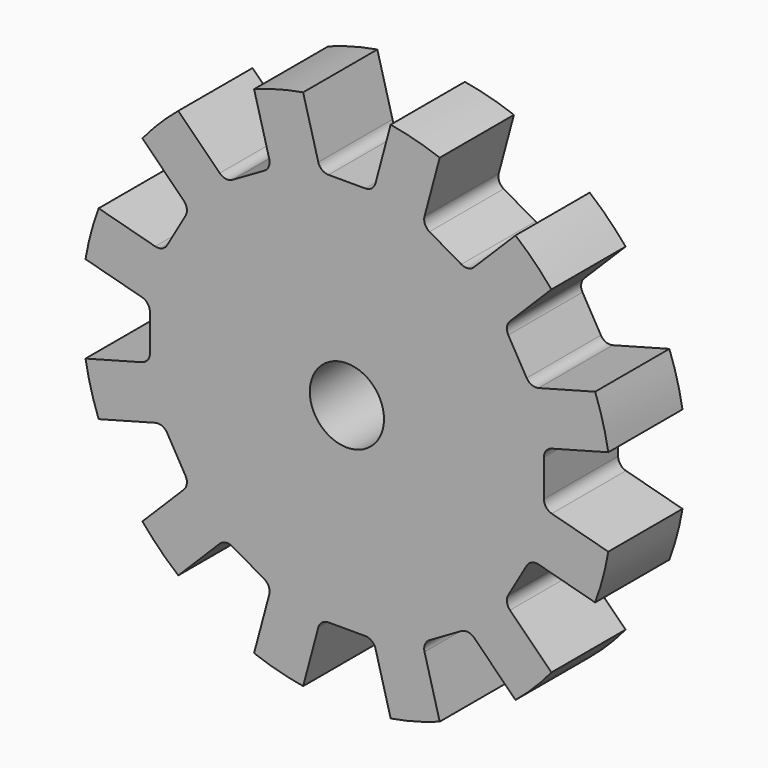
from build123d import *

# Parameters (mm, degrees)
F0_R     = 25.4
F1_DEPTH = 8.89
F3_DEPTH = 25.4
F4_COUNT = 12
F4_ANGLE = 330
F5_R     = 3.556
F6_DEPTH = 25.4


with BuildPart() as f1:
    # F0 (on Front) → F1 (new body)
    with BuildSketch(Plane.XZ):
        Circle(F0_R)
    extrude(amount=F1_DEPTH)

    # F2 (on face) → F3 (cut)
    with BuildSketch(Plane.XZ.offset(8.89)):
        with BuildLine():
            ThreePointArc((1.7603957802, 18.8799073091), (2.3788973921, 19.0898603154), (2.7417764197, 19.6329471593))
            Line((2.7417764197, 19.6329471593), (4.19365, 25.0514131273))
            ThreePointArc((4.19365, 25.0514131274), (0, 25.4), (-4.19365, 25.0514131274))
            Line((-4.19365, 25.0514131273), (-2.7417764197, 19.6329471593))
            ThreePointArc((-2.7417764197, 19.6329471593), (-2.3788973921, 19.0898603154), (-1.7603957802, 18.8799073091))
            Line((-1.7603957802, 18.8799073091), (0, 18.8799073091))
            Line((0, 18.8799073091), (1.7603957802, 18.8799073091))
        make_face()
    f3 = extrude(amount=-F3_DEPTH, mode=Mode.SUBTRACT)

    # F4: F3 ×12 about axis
    f4_axis = Axis((0, 0, 0), (0, 1, 0))
    for i in range(1, F4_COUNT):
        add(f3.rotate(f4_axis, i * F4_ANGLE / (F4_COUNT - 1)), mode=Mode.SUBTRACT)

    # F5 (on face) → F6 (cut)
    with BuildSketch(Plane.XZ.offset(8.89)):
        Circle(F5_R)
    extrude(amount=-F6_DEPTH, mode=Mode.SUBTRACT)


solid = f1.part
